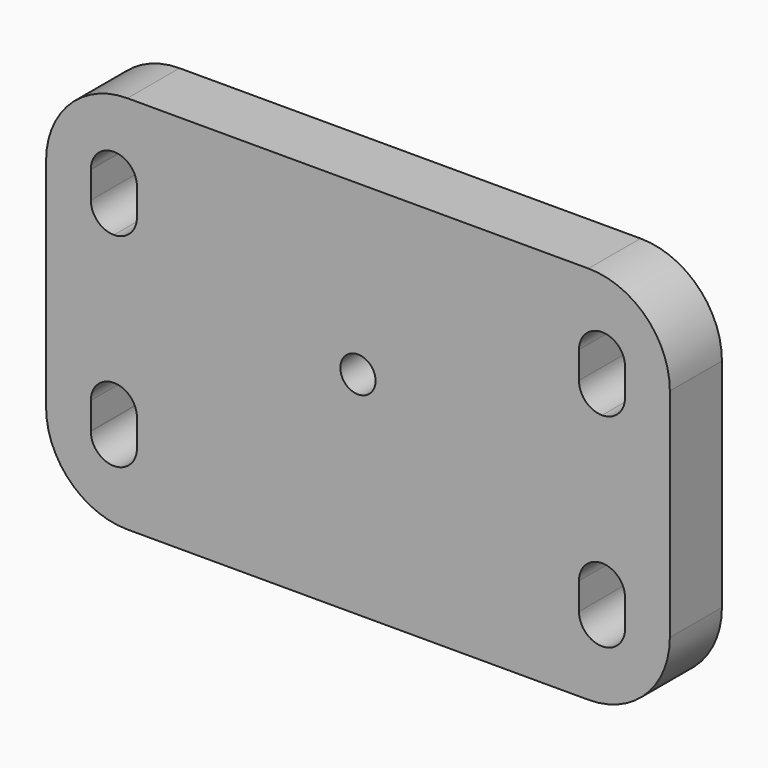
from build123d import *

# Parameters (mm, degrees)
F0_W     = 115
F0_H     = 70
F1_DEPTH = 12
F2_W     = 4.25
F2_H     = 5
F2_W_2   = 4.2500000007
F3_DEPTH = 25
F4_R     = 3.25
F5_DEPTH = 25
F6_R     = 15


with BuildPart() as f1:
    # F0 (on Front) → F1 (new body)
    with BuildSketch(Plane.XZ):
        Rectangle(F0_W, F0_H)
    extrude(amount=F1_DEPTH)

    # F2 (on face) → F3 (cut)
    with BuildSketch(Plane.XZ.offset(12)):
        with BuildLine():
            Line((-40.75, 16.25), (-40.75, 21.25))
            ThreePointArc((-40.75, 21.25), (-44.9763637107, 25.4999342731), (-49.2497370945, 21.2972718474))
            Line((-49.2497370945, 21.2972718474), (-49.2497419962, 21.2031708885))
            Line((-49.2497419962, 21.2031708885), (-49.2499999942, 16.2502213815))
            ThreePointArc((-49.2499999942, 16.2502213815), (-48.0052820892, 13.2448744512), (-45, 12))
            Line((-45, 12), (-45, 16.25))
            Line((-45, 16.25), (-40.75, 16.25))
        make_face()
        with BuildLine():
            ThreePointArc((49.2497370945, 21.2972718474), (44.9763637107, 25.4999342731), (40.75, 21.25))
            Line((40.75, 21.25), (40.75, 16.25))
            ThreePointArc((40.75, 16.25), (41.99479618, 19.25520382), (45, 20.5))
            ThreePointArc((45, 20.5), (46.9284060776, 20.0373143519), (48.4369317712, 18.75))
            ThreePointArc((48.4369317712, 18.75), (49.041590439, 17.5645519096), (49.2499999942, 16.2502213815))
            Line((49.2499999942, 16.2502213815), (49.2497419962, 21.2031708885))
            Line((49.2497419962, 21.2031708885), (49.2497370945, 21.2972718474))
        make_face()
        with BuildLine():
            ThreePointArc((-45, 12), (-41.99479618, 13.24479618), (-40.75, 16.25))
            Line((-40.75, 16.25), (-45, 16.25))
            Line((-45, 16.25), (-45, 12))
        make_face()
        with BuildLine():
            ThreePointArc((45, 20.5), (41.99479618, 19.25520382), (40.75, 16.25))
            Line((40.75, 16.25), (45, 16.25))
            Line((45, 16.25), (45, 20.5))
        make_face()
        with BuildLine():
            Line((45, 16.25), (40.75, 16.25))
            ThreePointArc((40.75, 16.25), (41.99479618, 13.24479618), (45, 12))
            Line((45, 12), (45, 16.25))
        make_face()
        with BuildLine():
            Line((45, 20.5), (45, 16.25))
            Line((45, 16.25), (45, 12))
            ThreePointArc((45, 12), (48.00520382, 13.24479618), (49.25, 16.25))
            ThreePointArc((49.25, 16.25), (49.2499999986, 16.2501106908), (49.2499999942, 16.2502213815))
            ThreePointArc((49.2499999942, 16.2502213815), (49.041590439, 17.5645519096), (48.4369317712, 18.75))
            ThreePointArc((48.4369317712, 18.75), (46.9284060776, 20.0373143519), (45, 20.5))
        make_face()
        with BuildLine():
            ThreePointArc((-40.75, -16.25), (-41.99479618, -13.24479618), (-45, -12))
            Line((-45, -12), (-45, -16.25))
            Line((-45, -16.25), (-40.75, -16.25))
        make_face()
        with BuildLine():
            Line((-45, -16.25), (-45, -12))
            ThreePointArc((-45, -12), (-48.0052820892, -13.2448744512), (-49.2499999942, -16.2502213815))
            Line((-49.2499999942, -16.2502213815), (-49.2497419962, -21.2031708885))
            Line((-49.2497419962, -21.2031708885), (-49.2497370945, -21.2972718474))
            ThreePointArc((-49.2497370945, -21.2972718474), (-44.9763637107, -25.4999342731), (-40.75, -21.25))
            Line((-40.75, -21.25), (-45, -21.25))
            Line((-45, -21.25), (-45, -16.25))
        make_face()
        with BuildLine():
            ThreePointArc((49.2499999957, -16.2502213815), (48.005242953, -13.2449460071), (45, -12.0001106908))
            Line((45, -12.0001106908), (45, -16.25))
            Line((45, -16.25), (45, -21.25))
            Line((45, -21.25), (40.75, -21.25))
            ThreePointArc((40.75, -21.25), (44.9763637107, -25.4999342731), (49.2497370945, -21.2972718474))
            Line((49.2497370945, -21.2972718474), (49.2497419962, -21.2031708885))
            Line((49.2497419962, -21.2031708885), (49.2499999942, -16.2502213815))
        make_face()
        with BuildLine():
            Line((45, -16.25), (45, -12.0001106908))
            ThreePointArc((45, -12.0001106908), (41.9948353134, -13.2448677349), (40.7499999986, -16.25))
            Line((40.7499999993, -16.25), (45, -16.25))
        make_face()
        with Locations((-42.875, -18.75)):
            Rectangle(F2_W, F2_H)
        with Locations((42.8749999996, -18.75)):
            Rectangle(F2_W_2, F2_H)
    extrude(amount=-F3_DEPTH, mode=Mode.SUBTRACT)

    # F4 (on face) → F5 (cut)
    with BuildSketch(Plane.XZ.offset(12)):
        with Locations((0, 4)):
            Circle(F4_R)
    extrude(amount=-F5_DEPTH, mode=Mode.SUBTRACT)

    # F6
    f6_edges = [f1.edges().sort_by_distance(p)[0] for p in [
        (-57.5, -6, 35),
        (57.5, -6, 35),
        (57.5, -6, -35),
        (-57.5, -6, -35),
    ]]
    fillet(f6_edges, radius=F6_R)


solid = f1.part
